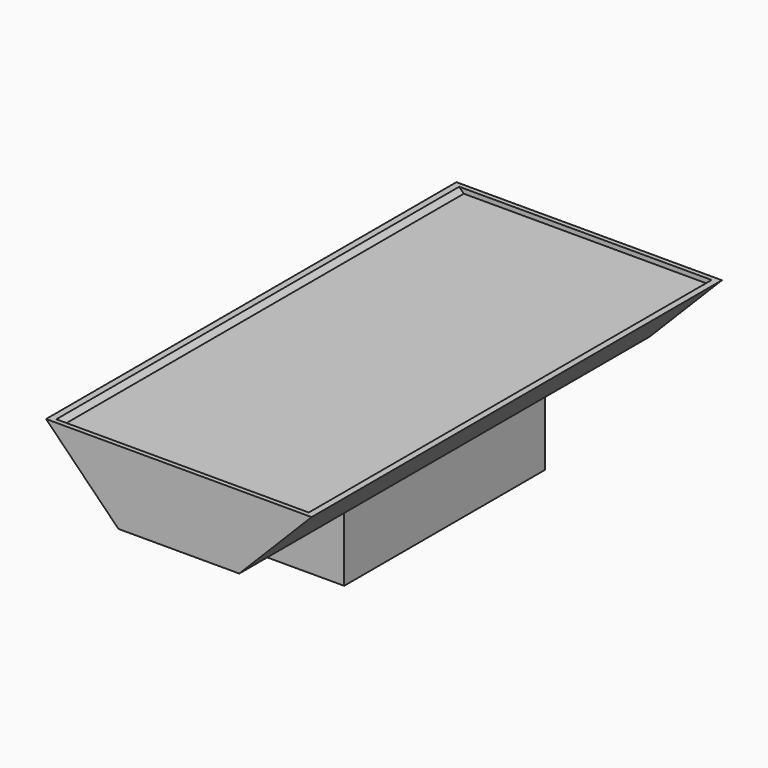
from build123d import *

# Parameters (mm, degrees)
F1_DEPTH     = 140.081
F2_DEPTH     = 140.0048
F3_DEPTH     = 68.5038
F4_DEPTH     = 68.5038
F5_T         = -5.08
F6_T         = 2.54
F6_T3_DEPTH  = 142.0876
F6_T5_DEPTH  = 71.08
F6_T7_DEPTH  = 275.0058
F6_T9_DEPTH  = 47.0194652776
F6_T11_DEPTH = 76.581
F6_T13_DEPTH = 9.2884577092
F6_T15_DEPTH = 76.6572
F6_T17_DEPTH = 125.7681103512
F6_T19_DEPTH = 47.0149573841
F6_T21_DEPTH = 66.8341103512
F6_T23_DEPTH = 47.0149573841
F6_T25_DEPTH = 9.2884593969
F6_T27_DEPTH = 42.1653521873
F6_T29_DEPTH = 42.16567527


# Not quite as in the source:
# - a shell that OpenCascade refuses in one call is made with other operations: the cavity is built on its own and cut out


with BuildPart() as f1:
    # F0 (on Front) → F1 (new body)
    with BuildSketch(Plane.XZ):
        Polygon((-72.5043, 57.5), (-33, 17.5), (0, 17.5), (33, 17.5), (72.4957, 57.5), align=None)
    extrude(amount=F1_DEPTH)

    # F0 (on Front) → F2 (join)
    with BuildSketch(Plane.XZ):
        Polygon((-72.5043, 57.5), (-33, 17.5), (0, 17.5), (33, 17.5), (72.4957, 57.5), align=None)
    extrude(amount=-F2_DEPTH)

    # F0 (on Front) → F3 (join)
    with BuildSketch(Plane.XZ):
        Polygon((-33, 17.5), (-33, -17.5), (33, -17.5), (33, 17.5), (0, 17.5), align=None)
    extrude(amount=-F3_DEPTH)

    # F0 (on Front) → F4 (join)
    with BuildSketch(Plane.XZ):
        Polygon((-33, 17.5), (-33, -17.5), (33, -17.5), (33, 17.5), (0, 17.5), align=None)
    extrude(amount=F4_DEPTH)

    # F5
    f5_openings = [f1.faces().sort_by_distance(p)[0] for p in [
        (0, 0, -17.5),
    ]]
    offset(amount=F5_T, openings=f5_openings, kind=Kind.INTERSECTION)

    # F6: shell of thickness 2.54, made by hand


with BuildPart() as f6_core1:
    # F6_t2: copy of F1
    add(f1.part)

    # the walls: a layer under each face that stays
    f6_faces = [f6_core1.faces().sort_by_distance(p)[0] for p in [
        (-52.75215, -0.0381, 37.5),
        (-0.0043, 140.0048, 37.5),
        (52.74785, -0.0381, 37.5),
        (33, 0, 0),
        (0, -68.5038, 0),
        (0, 68.5038, 0),
        (0, 104.2543, 17.5),
        (-33, 0, 0),
        (0, -104.2924, 17.5),
        (-0.0043, -140.081, 37.5),
        (-28.2857142857, 58.7175428571, -17.5),
        (-44.1337126804, -0.0381, 36.002837635),
        (-0.0033701852, 134.9248, 37.5),
        (44.1303424952, -0.0381, 36.0026760937),
        (27.92, 0, 1.0426760937),
        (28.4128154651, -63.4238, 21.0826760937),
        (0, -63.4238, 2.54),
        (-29.3986087804, -63.4238, 22.0809458783),
        (28.4128154651, 63.4238, 21.0826760937),
        (0, 63.4238, 2.54),
        (-29.3986087804, 63.4238, 22.0809458783),
        (-0.0001623852, 99.1743, 22.58),
        (-27.92, 0, 1.042837635),
        (-0.0001623852, -99.2124, 22.58),
        (-0.0033701852, -135.001, 37.5),
        (-0.0033701852, -0.0381, 52.42),
    ]]
    thicken(f6_faces, amount=-F6_T, mode=Mode.SUBTRACT)

    # F6_s4 → F6_t3 (cut)
    with BuildSketch(Plane.XZ.offset(-71.0438)):
        Polygon((-33.0434721427, 17.4821518164), (-31.192785733, 19.2848183642), (-30.46, 18.542837635), (-30.46, 17.5), align=None)
        Polygon((33.0434740854, 17.4821537837), (31.1925914624, 19.2846216345), (30.46, 18.5426760937), (30.46, 17.5), align=None)
    extrude(amount=F6_T3_DEPTH, mode=Mode.SUBTRACT)

    # F6_s6 → F6_t5 (cut)
    with BuildSketch(Plane.YZ.offset(-35.54)):
        Polygon((-68.5292, 17.4746), (-65.9638, 17.5), (-65.9638, 20.04), (-68.5038, 20.04), align=None)
        Polygon((68.5292, 17.4746), (65.9638, 17.5), (65.9638, 20.04), (68.5038, 20.04), align=None)
    extrude(amount=F6_T5_DEPTH, mode=Mode.SUBTRACT)

    # F6_s8 → F6_t7 (cut)
    with BuildSketch(Plane.XZ.offset(-137.4648)):
        Polygon((-60.3293532181, 52.4124481836), (-62.1546396278, 50.6351816358), (-66.4258626804, 54.96), (-60.3474253608, 54.96), align=None)
        Polygon((60.322610905, 52.4124462163), (62.148093528, 50.6353783655), (66.4181924952, 54.96), (60.3406849904, 54.96), align=None)
    extrude(amount=F6_T7_DEPTH, mode=Mode.SUBTRACT)

    # F6_s10 → F6_t9 (cut)
    with BuildSketch(Plane(origin=(-57.7902488571, 0, 58.5154009635), x_dir=(0, 1, 0), z_dir=(0.7026843954, 0, -0.7115016799))):
        Polygon((134.8994, -6.0771785187), (134.9248, -8.6425785187), (137.4648, -8.6425785187), (137.4648, -6.1025785187), align=None)
        Polygon((-134.9756, -6.0771785187), (-135.001, -8.6425785187), (-137.541, -8.6425785187), (-137.541, -6.1025785187), align=None)
    extrude(amount=F6_T9_DEPTH, mode=Mode.SUBTRACT)

    # F6_s12 → F6_t11 (cut)
    with BuildSketch(Plane.XZ.offset(-137.4648)):
        Polygon((-30.8591454181, 22.6232481836), (-32.6844318278, 20.7951816358), (-31.9386087804, 20.04), (-30.8772175608, 20.04), align=None)
        Polygon((30.858818705, 22.6232462163), (32.684301328, 20.7953783655), (31.9384463952, 20.04), (30.8768927904, 20.04), align=None)
    extrude(amount=F6_T11_DEPTH, mode=Mode.SUBTRACT)

    # F6_s14 → F6_t13 (cut)
    with BuildSketch(Plane(origin=(-28.3200410571, 0, 28.6754009635), x_dir=(0, 1, 0), z_dir=(0.7026843954, 0, -0.7115016799))):
        Polygon((63.3984, -6.0771785187), (63.4238, -8.6425785187), (65.9638, -8.6425785187), (65.9638, -6.1025785187), align=None)
        Polygon((-63.3984, -6.0771785187), (-63.4238, -8.6425785187), (-65.9638, -8.6425785187), (-65.9638, -6.1025785187), align=None)
    extrude(amount=F6_T13_DEPTH, mode=Mode.SUBTRACT)

    # F6_s16 → F6_t15 (cut)
    with BuildSketch(Plane.XZ.offset(60.8838)):
        Polygon((-30.8591454181, 22.6232481836), (-32.6844318278, 20.7951816358), (-31.9386087804, 20.04), (-30.8772175608, 20.04), align=None)
        Polygon((30.858818705, 22.6232462163), (32.684301328, 20.7953783655), (31.9384463952, 20.04), (30.8768927904, 20.04), align=None)
    extrude(amount=F6_T15_DEPTH, mode=Mode.SUBTRACT)

    # F6_s18 → F6_t17 (cut)
    with BuildSketch(Plane.YZ.offset(-62.8874253608)):
        Polygon((134.8994, 52.3946), (137.4648, 52.42), (137.4648, 54.96), (134.9248, 54.96), align=None)
        Polygon((-134.9756, 52.3946), (-137.541, 52.42), (-137.541, 54.96), (-135.001, 54.96), align=None)
    extrude(amount=F6_T17_DEPTH, mode=Mode.SUBTRACT)

    # F6_s20 → F6_t19 (cut)
    with BuildSketch(Plane(origin=(57.7800845012, 0, 58.5178482733), x_dir=(0, 1, 0), z_dir=(-0.7026069427, 0, -0.7115781644))):
        Polygon((134.8994, 6.0810579283), (137.4648, 6.1064579283), (137.4648, 8.6464579283), (134.9248, 8.6464579283), align=None)
    extrude(amount=F6_T19_DEPTH, mode=Mode.SUBTRACT)

    # F6_s22 → F6_t21 (cut)
    with BuildSketch(Plane.YZ.offset(-33.4172175608)):
        Polygon((134.8994, 22.6054), (137.4648, 22.58), (137.4648, 20.04), (134.9248, 20.04), align=None)
        Polygon((-134.9756, 22.6054), (-135.001, 20.04), (-137.541, 20.04), (-137.541, 22.58), align=None)
    extrude(amount=F6_T21_DEPTH, mode=Mode.SUBTRACT)

    # F6_s24 → F6_t23 (cut)
    with BuildSketch(Plane(origin=(24.7470490323, 0, 25.0630311981), x_dir=(0, 1, 0), z_dir=(0.7026069427, 0, 0.7115781644))):
        Polygon((-134.9756, -6.0810579283), (-135.001, -8.6464579283), (-137.541, -8.6464579283), (-137.541, -6.1064579283), align=None)
    extrude(amount=F6_T23_DEPTH, mode=Mode.SUBTRACT)

    # F6_s26 → F6_t25 (cut)
    with BuildSketch(Plane(origin=(21.7901562419, 0, 22.0683833854), x_dir=(0, 1, 0), z_dir=(0.7026069427, 0, 0.7115781644))):
        Polygon((-63.3984, -6.0810579283), (-63.4238, -8.6464579283), (-65.9638, -8.6464579283), (-65.9638, -6.1064579283), align=None)
        Polygon((63.3984, -6.0810579283), (63.4238, -8.6464579283), (65.9638, -8.6464579283), (65.9638, -6.1064579283), align=None)
    extrude(amount=F6_T25_DEPTH, mode=Mode.SUBTRACT)

    # F6_s28 → F6_t27 (cut)
    with BuildSketch(Plane.XY.offset(-20.04)):
        Polygon((27.8946, 63.3984), (30.46, 63.4238), (30.46, 65.9638), (27.92, 65.9638), align=None)
        Polygon((27.8946, -63.3984), (30.46, -63.4238), (30.46, -65.9638), (27.92, -65.9638), align=None)
    extrude(amount=F6_T27_DEPTH, mode=Mode.SUBTRACT)

    # F6_s30 → F6_t29 (cut)
    with BuildSketch(Plane.XY.offset(-20.04)):
        Polygon((-27.8946, -63.3984), (-27.92, -65.9638), (-30.46, -65.9638), (-30.46, -63.4238), align=None)
        Polygon((-27.8946, 63.3984), (-27.92, 65.9638), (-30.46, 65.9638), (-30.46, 63.4238), align=None)
    extrude(amount=F6_T29_DEPTH, mode=Mode.SUBTRACT)


with BuildPart() as f1_1:
    add(f1.part)

    # what is left inside the walls is the cavity
    f6_cavity = [f6_core1.part.solids().sort_by_distance(p)[0] for p in [
        (-0.004108, -45.8724, 57.4746),
    ]]
    add(f6_cavity, mode=Mode.SUBTRACT)


solid = f1_1.part
